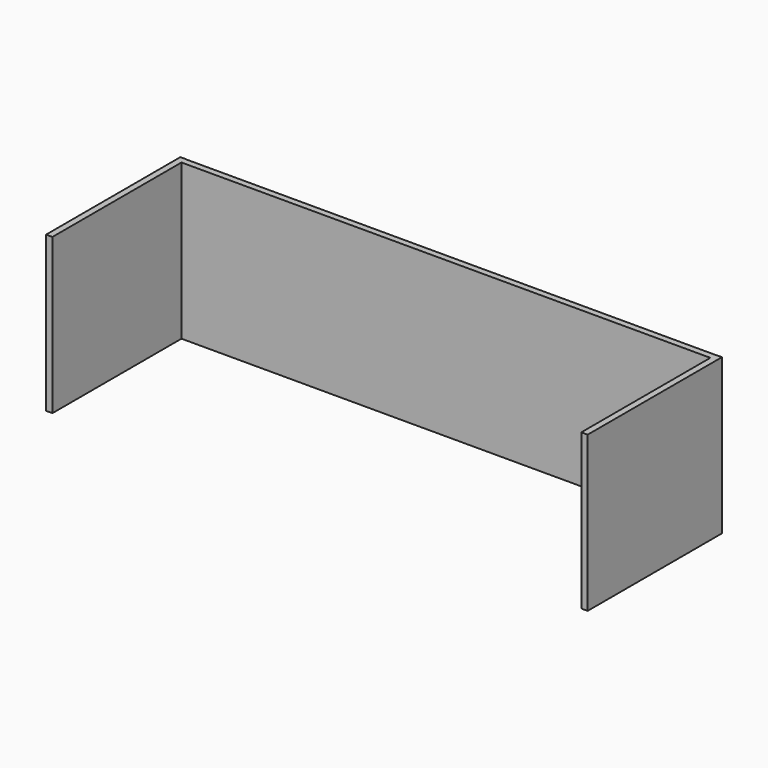
from build123d import *

# Parameters (mm, degrees)
F0_W     = 2381.25
F0_H     = 28.575
F1_DEPTH = 698.5
F3_W     = 0.762
F3_H     = 698.5
F3_W_2   = 28.575
F3_W_3   = 726.313
F4_DEPTH = 28.575
F2_W     = 726.313
F2_H     = 698.5
F2_W_2   = 28.575
F2_W_3   = 0.762
F5_DEPTH = 28.575


with BuildPart() as f1:
    # F0 (on Top) → F1 (new body)
    with BuildSketch(Plane.XY):
        with Locations((933.8365292177, 70.3620000839)):
            Rectangle(F0_W, F0_H)
    extrude(amount=F1_DEPTH)

    # F3 (on face) → F4 (join)
    with BuildSketch(Plane(origin=(-256.7884707823, 0, 0), x_dir=(0, -1, 0), z_dir=(-1, 0, 0))):
        with Locations((-85.0305000839, 349.25)):
            Rectangle(F3_W, F3_H)
        with Locations((-70.3620000839, 349.25)):
            Rectangle(F3_W_2, F3_H)
        with Locations((307.0819999161, 349.25)):
            Rectangle(F3_W_3, F3_H)
    extrude(amount=F4_DEPTH)

    # F2 (on face) → F5 (join)
    with BuildSketch(Plane.YZ.offset(2124.4615292177)):
        with Locations((-307.0819999161, 349.25)):
            Rectangle(F2_W, F2_H)
        with Locations((70.3620000839, 349.25)):
            Rectangle(F2_W_2, F2_H)
        with Locations((85.0305000839, 349.25)):
            Rectangle(F2_W_3, F2_H)
    extrude(amount=F5_DEPTH)


solid = f1.part
